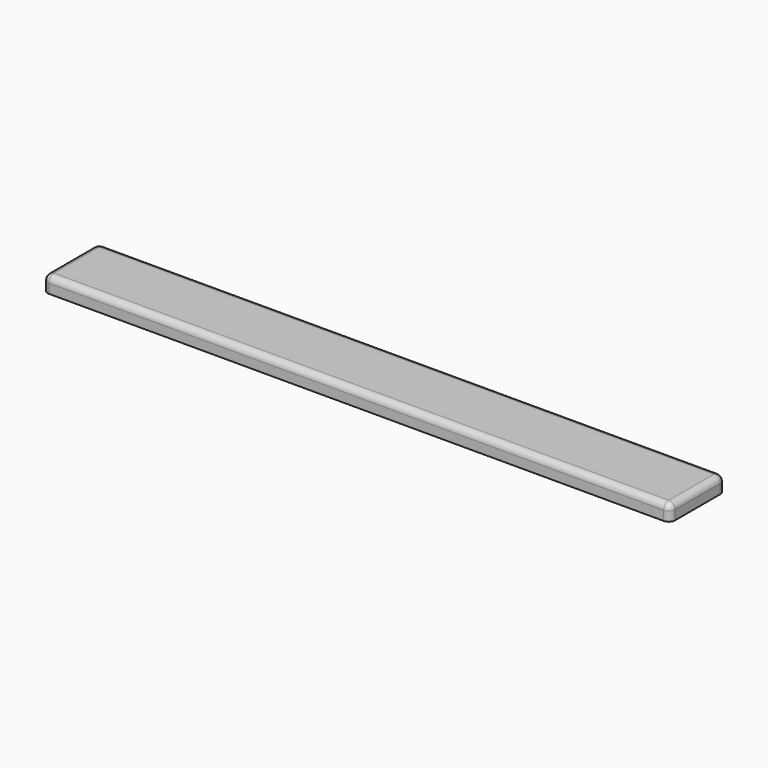
from build123d import *

# Parameters (mm, degrees)
F1_DEPTH = 1000
F2_R     = 10


with BuildPart() as f1:
    # F0 (on Right) → F1 (new body)
    with BuildSketch(Plane.YZ):
        with BuildLine():
            Line((-55, -12.5), (55, -12.5))
            Line((55, -12.5), (55, 2.5))
            ThreePointArc((55, 2.5), (52.0710678119, 9.5710678119), (45, 12.5))
            Line((45, 12.5), (-45, 12.5))
            ThreePointArc((-45, 12.5), (-52.0710678119, 9.5710678119), (-55, 2.5))
            Line((-55, 2.5), (-55, -12.5))
        make_face()
    extrude(amount=F1_DEPTH)

    # F2
    f2_edges = [f1.edges().sort_by_distance(p)[0] for p in [
        (1000, 0, 12.5),
        (500, 45, 12.5),
        (500, -45, 12.5),
        (0, 0, 12.5),
    ]]
    fillet(f2_edges, radius=F2_R)


solid = f1.part
